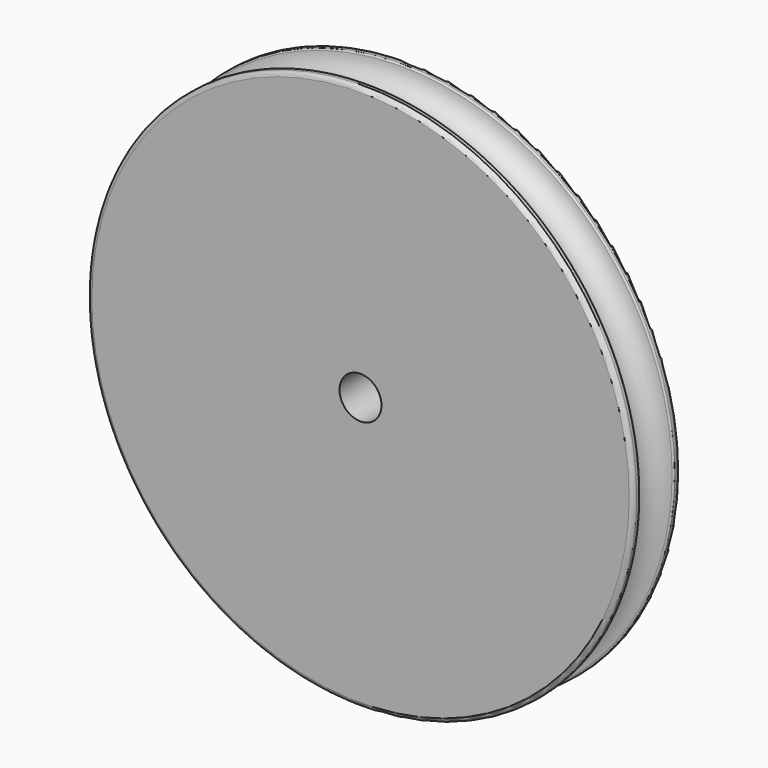
from build123d import *

# Parameters (mm, degrees)
F2_R     = 0.635
F3_R     = 0.254
F4_R     = 3.175
F5_DEPTH = 8.891


with BuildPart() as f1:
    # F0 (on Top) → F1 (revolve)
    with BuildSketch(Plane.XY):
        with BuildLine():
            Line((41.275, 4.445), (0, 4.445))
            Line((0, 4.445), (0, -4.445))
            Line((0, -4.445), (41.275, -4.445))
            Line((41.275, -4.445), (41.275, -3.175))
            ThreePointArc((41.275, -3.175), (38.1, 0), (41.275, 3.175))
            Line((41.275, 3.175), (41.275, 4.445))
        make_face()
    revolve(axis=Axis((0, 0, 0), (0, -1, 0)))

    # F2
    f2_edges = [f1.edges().sort_by_distance(p)[0] for p in [
        (-41.275, 4.445, 0),
        (-41.275, -4.445, 0),
    ]]
    fillet(f2_edges, radius=F2_R)

    # F3
    f3_edges = [f1.edges().sort_by_distance(p)[0] for p in [
        (-41.275, 3.175, 0),
        (-41.275, -3.175, 0),
    ]]
    fillet(f3_edges, radius=F3_R)

    # F4 (on face) → F5 (cut, through all)
    with BuildSketch(Plane.XZ.offset(4.445)):
        Circle(F4_R)
    extrude(amount=-F5_DEPTH, mode=Mode.SUBTRACT)


solid = f1.part
